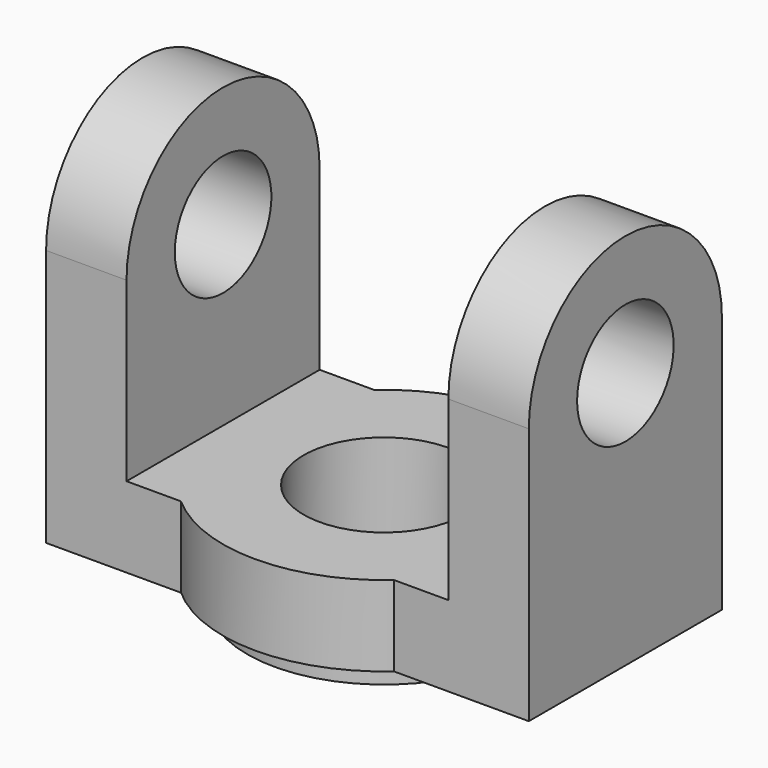
from build123d import *

# Parameters (mm, degrees)
F0_W     = 60
F0_H     = 30
F0_R     = 10
F1_DEPTH = 10
F2_R     = 10
F3_DEPTH = 10
F4_R     = 17
F4_R_2   = 10
F5_DEPTH = 3
F7_DEPTH = 60
F8_W     = 40
F8_H     = 41
F9_DEPTH = 35.001


with BuildPart() as f1:
    # F0 (on Top) → F1 (new body)
    with BuildSketch(Plane.XY):
        with Locations((30, 15)):
            Rectangle(F0_W, F0_H)
        with Locations((30, 15)):
            Circle(F0_R, mode=Mode.SUBTRACT)
    extrude(amount=F1_DEPTH)

    # F2 (on face) → F3 (join)
    with BuildSketch(Plane.XY.offset(10)):
        with BuildLine():
            ThreePointArc((43.2287565553, 0), (48.2287565553, 6.7712434447), (50, 15))
            ThreePointArc((50, 15), (48.2287565553, 23.2287565553), (43.2287565553, 30))
            Line((43.2287565553, 30), (16.7712434447, 30))
            ThreePointArc((16.7712434447, 30), (11.7712434447, 23.2287565553), (10, 15))
            ThreePointArc((10, 15), (11.7712434447, 6.7712434447), (16.7712434447, 0))
            Line((16.7712434447, 0), (43.2287565553, 0))
        make_face()
        with Locations((30, 15)):
            Circle(F2_R, mode=Mode.SUBTRACT)
        with BuildLine():
            Line((16.7712434447, 30), (43.2287565553, 30))
            ThreePointArc((43.2287565553, 30), (30, 35), (16.7712434447, 30))
        make_face()
        with BuildLine():
            ThreePointArc((16.7712434447, 0), (30, -5), (43.2287565553, 0))
            Line((43.2287565553, 0), (16.7712434447, 0))
        make_face()
    extrude(amount=-F3_DEPTH)

    # F4 (on face) → F5 (join)
    with BuildSketch(Plane(origin=(0, 0, 0), x_dir=(1, 0, 0), z_dir=(0, 0, -1))):
        with Locations((30, -15)):
            Circle(F4_R)
        with Locations((30, -15)):
            Circle(F4_R_2, mode=Mode.SUBTRACT)
    extrude(amount=F5_DEPTH)

    # F6 (on face) → F7 (join, through all)
    with BuildSketch(Plane.YZ.offset(60)):
        with BuildLine():
            Line((0, 32), (0, 10))
            Line((0, 10), (30, 10))
            Line((30, 10), (30, 32))
            Line((30, 32), (22.5, 32))
            ThreePointArc((22.5, 32), (15, 24.5), (7.5, 32))
            Line((7.5, 32), (0, 32))
        make_face()
        with BuildLine():
            ThreePointArc((30, 32), (15, 47), (0, 32))
            Line((0, 32), (7.5, 32))
            ThreePointArc((7.5, 32), (15, 39.5), (22.5, 32))
            Line((22.5, 32), (30, 32))
        make_face()
    extrude(amount=-F7_DEPTH)

    # F8 (on Front) → F9 (cut, through all)
    with BuildSketch(Plane.XZ):
        with Locations((29.9999999726, 30.5)):
            Rectangle(F8_W, F8_H)
    extrude(amount=-F9_DEPTH, mode=Mode.SUBTRACT)


solid = f1.part
